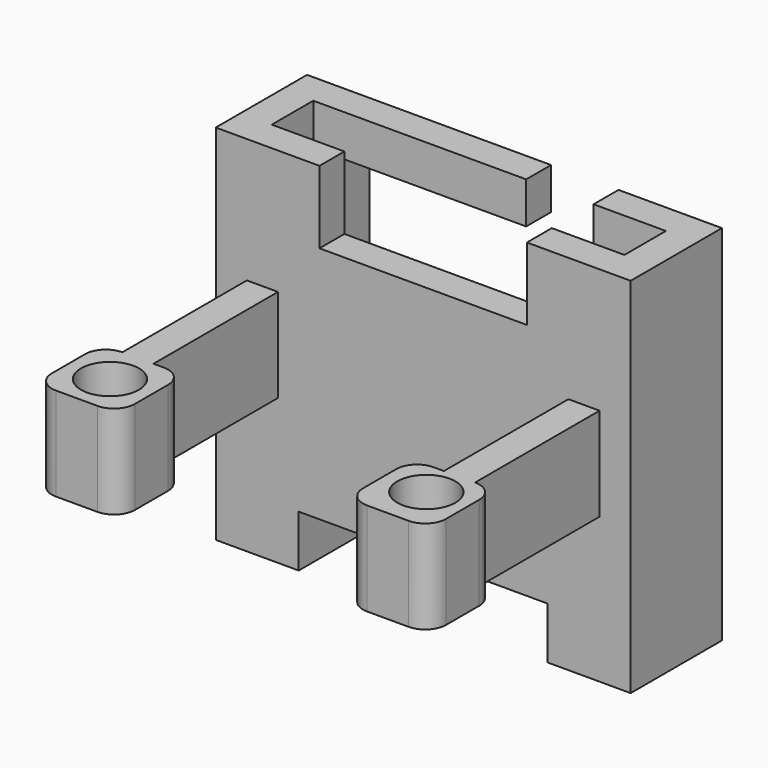
from build123d import *

# Parameters (mm, degrees)
F1_DEPTH  = 1.5
F2_W      = 3
F2_H      = 9
F3_DEPTH  = 15
F4_W      = 2
F4_H      = 9
F5_DEPTH  = 8
F7_D      = 5.6
F8_R      = 1.99999
F9_W      = 5
F9_H      = 3
F10_DEPTH = 3
F12_DEPTH = 2
F13_DEPTH = 2
F14_W     = 3
F14_H     = 4
F14_W_2   = 2
F14_H_2   = 3
F14_W_3   = 9.8253687732
F14_H_3   = 5
F15_DEPTH = 3
F16_W     = 6.5
F16_H     = 4
F17_DEPTH = 3


# Not quite as in the source:
# - a fillet or chamfer is up to 0.001 mm smaller than in the source, because OpenCascade refuses the exact size


with BuildPart() as f1:
    # F0 (on Front) → F1 (new body, symmetric)
    with BuildSketch(Plane.XZ):
        Polygon((-46.7140089311, 21.8801796436), (-46.7140089311, 6.5596503988), (-41.7140089311, 6.5596503988), (-41.7140089311, 8.5596503988), (-29.7140089311, 8.5596503988), (-29.7140089311, 21.8801796436), align=None)
        Polygon((-46.7140089311, 38.5596503988), (-46.7140089311, 21.8801796436), (-29.7140089311, 21.8801796436), (-29.7140089311, 31.5596503988), (-39.7140089311, 31.5596503988), (-39.7140089311, 38.5596503988), align=None)
        Polygon((-12.7140089311, 21.8801796436), (-29.7140089311, 21.8801796436), (-29.7140089311, 8.5596503988), (-17.7140089311, 8.5596503988), (-17.7140089311, 6.5596503988), (-12.7140089311, 6.5596503988), align=None)
        Polygon((-29.7140089311, 31.5596503988), (-29.7140089311, 21.8801796436), (-12.7140089311, 21.8801796436), (-12.7140089311, 38.5596503988), (-19.7140089311, 38.5596503988), (-19.7140089311, 31.5596503988), align=None)
    extrude(amount=F1_DEPTH, both=True)

    # F2 (on face) → F3 (join)
    with BuildSketch(Plane.XZ.offset(1.5)):
        with Locations((-45.2140089311, 22.0596503988)):
            Rectangle(F2_W, F2_H)
        with Locations((-14.2140089311, 22.0596503988)):
            Rectangle(F2_W, F2_H)
    extrude(amount=F3_DEPTH)

    # F4 (on face) → F5 (join)
    with BuildSketch(Plane.XZ.offset(16.5)):
        Polygon((-44.7140089311, 26.5596503988), (-46.7140089311, 26.5596503988), (-46.7140089311, 17.5596503988), (-43.7140089311, 17.5596503988), (-40.7140089311, 17.5596503988), (-40.7140089311, 26.5596503988), (-43.7140089311, 26.5596503988), align=None)
        with Locations((-47.7140089311, 22.0596503988)):
            Rectangle(F4_W, F4_H)
        Polygon((-12.7140089311, 17.5596503988), (-12.7140089311, 26.5596503988), (-14.7140089311, 26.5596503988), (-15.7140089311, 26.5596503988), (-18.7140089311, 26.5596503988), (-18.7140089311, 17.5596503988), (-15.7140089311, 17.5596503988), align=None)
        with Locations((-11.7140089311, 22.0596503988)):
            Rectangle(F4_W, F4_H)
    extrude(amount=F5_DEPTH)

    # F7 (through all)
    with Locations(Plane.XY.offset(26.5596503988)):
        with Locations((-44.7140089311, -20.5), (-14.6104083322, -20)):
            Hole(F7_D / 2)

    # F8 (radius 2 in the source; OpenCascade refuses exactly that, so slightly less here)
    f8_edges = [f1.edges().sort_by_distance(p)[0] for p in [
        (-10.714009, -16.5, 22.05965),
        (-18.714009, -16.5, 22.05965),
        (-18.714009, -24.5, 22.05965),
        (-10.714009, -24.5, 22.05965),
        (-48.714009, -24.5, 22.05965),
        (-48.714009, -16.5, 22.05965),
        (-40.714009, -16.5, 22.05965),
        (-40.714009, -24.5, 22.05965),
    ]]
    fillet(f8_edges, radius=F8_R)

    # F9 (on face) → F10 (join, symmetric)
    with BuildSketch(Plane(origin=(0, 1.5, 0), x_dir=(-1, 0, 0), z_dir=(0, 1, 0))):
        Polygon((12.7140089311, 6.5596503988), (12.7140089311, 38.5596503988), (9.7140089311, 38.5596503988), (9.7140089311, 3.5596503988), (12.7140089311, 3.5596503988), align=None)
        with Locations((15.2140089311, 5.0596503988)):
            Rectangle(F9_W, F9_H)
        with Locations((44.2140089311, 5.0596503988)):
            Rectangle(F9_W, F9_H)
        Polygon((49.7140089311, 38.5596503988), (46.7140089311, 38.5596503988), (46.7140089311, 6.5596503988), (46.7140089311, 3.5596503988), (49.7140089311, 3.5596503988), align=None)
    extrude(amount=F10_DEPTH, both=True)

    # F11 (on face) → F12 (join)
    with BuildSketch(Plane(origin=(0, 4.5, 0), x_dir=(-1, 0, 0), z_dir=(0, 1, 0))):
        Polygon((49.7140089311, 3.5596503988), (49.7140089311, 38.5596503988), (46.7140089311, 38.5596503988), (46.7140089311, 6.5596503988), (41.7140089311, 6.5596503988), (41.7140089311, 3.5596503988), align=None)
    extrude(amount=F12_DEPTH)

    # F13 (add): a face of the model
    f13_faces = [f1.faces().sort_by_distance(p)[0] for p in [
        (-11.7140089311, 4.5, 19.0596503988),
    ]]
    extrude(f13_faces, amount=F13_DEPTH)

    # F14 (on face) → F15 (join)
    with BuildSketch(Plane(origin=(0, 6.5, 0), x_dir=(-1, 0, 0), z_dir=(0, 1, 0))):
        with Locations((48.2140089311, 36.5596503988)):
            Rectangle(F14_W, F14_H)
        Polygon((46.7140089311, 34.5596503988), (46.7140089311, 38.5596503988), (9.7140089311, 38.5596503988), (9.7140089311, 34.5596503988), (15.7140089311, 34.5596503988), (43.7140089311, 34.5596503988), align=None)
        Polygon((49.7140089311, 3.5596503988), (49.7140089311, 34.5596503988), (46.7140089311, 34.5596503988), (46.7140089311, 6.5596503988), (43.7140089311, 6.5596503988), (43.7140089311, 3.5596503988), align=None)
        Polygon((46.7140089311, 6.5596503988), (46.7140089311, 34.5596503988), (43.7140089311, 34.5596503988), (43.7140089311, 8.5596503988), (43.7140089311, 6.5596503988), align=None)
        Polygon((15.7140089311, 34.5596503988), (9.7140089311, 34.5596503988), (9.7140089311, 3.5596503988), (15.7140089311, 3.5596503988), (15.7140089311, 8.5596503988), align=None)
        with Locations((42.7140089311, 5.0596503988)):
            Rectangle(F14_W_2, F14_H_2)
        Polygon((43.7140089311, 6.5596503988), (43.7140089311, 8.5596503988), (33.8886401579, 8.5596503988), (33.8886401579, 3.5596503988), (41.7140089311, 3.5596503988), (41.7140089311, 6.5596503988), align=None)
        with Locations((20.6266933177, 6.0596503988)):
            Rectangle(F14_W_3, F14_H_3)
    extrude(amount=F15_DEPTH)

    # F16 (on face) → F17 (cut)
    with BuildSketch(Plane(origin=(0, 9.5, 0), x_dir=(-1, 0, 0), z_dir=(0, 1, 0))):
        with Locations((22.9359017015, 36.5596503988)):
            Rectangle(F16_W, F16_H)
    extrude(amount=-F17_DEPTH, mode=Mode.SUBTRACT)


solid = f1.part
